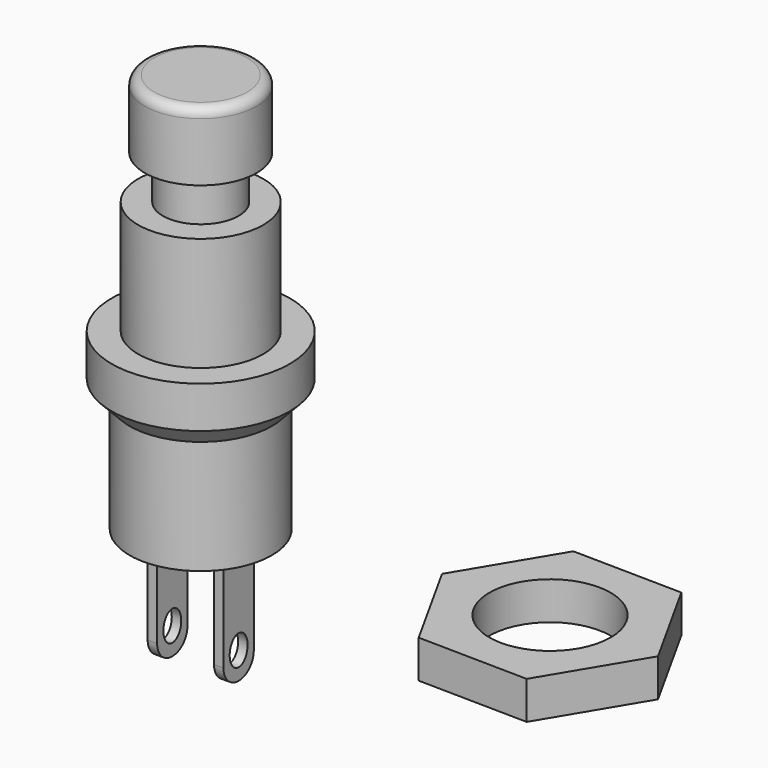
from build123d import *

# Parameters (mm, degrees)
F0_R      = 3.75
F0_W      = 0.5
F0_H      = 2
F1_DEPTH  = 6
F3_R      = 4.7
F1_FACE_R = 3.75
F5_DEPTH  = 2.2
F6_R      = 3.3
F7_DEPTH  = 6
F8_R      = 2
F9_DEPTH  = 2.3
F10_R     = 2.95
F11_DEPTH = 3.6
F12_R     = 0.5
F13_DEPTH = 6.4
F15_DEPTH = 6.7010001
F16_R     = 0.99999
F0_R_2    = 3.2
F17_DEPTH = 2


# Not quite as in the source:
# - a fillet or chamfer is up to 0.001 mm smaller than in the source, because OpenCascade refuses the exact size


with BuildPart() as f1:
    # F0 (on Top) → F1 (new body)
    with BuildSketch(Plane.XY):
        Circle(F0_R)
        with Locations((-1.75, 0)):
            Rectangle(F0_W, F0_H, mode=Mode.SUBTRACT)
        with Locations((1.75, 0)):
            Rectangle(F0_W, F0_H, mode=Mode.SUBTRACT)
        with Locations((-1.75, 0)):
            Rectangle(F0_W, F0_H)
        with Locations((1.75, 0)):
            Rectangle(F0_W, F0_H)
    extrude(amount=F1_DEPTH)

    # F3 (on offset) → F4 section 0
    with BuildSketch(Plane.XY.offset(7)):
        Circle(F3_R)
    # F1_face (on face) → F4 section 1
    with BuildSketch(Plane.XY.offset(6)):
        Circle(F1_FACE_R)
    loft()

    # F3 (on offset) → F5 (join)
    with BuildSketch(Plane.XY.offset(7)):
        Circle(F3_R)
    extrude(amount=F5_DEPTH)

    # F6 (on face) → F7 (join)
    with BuildSketch(Plane.XY.offset(9.2)):
        Circle(F6_R)
    extrude(amount=F7_DEPTH)

    # F8 (on face) → F9 (join)
    with BuildSketch(Plane.XY.offset(15.2)):
        Circle(F8_R)
    extrude(amount=F9_DEPTH)

    # F0 (on Top) → F13 (join)
    with BuildSketch(Plane.XY):
        with Locations((-1.75, 0)):
            Rectangle(F0_W, F0_H)
        with Locations((1.75, 0)):
            Rectangle(F0_W, F0_H)
    extrude(amount=-F13_DEPTH)

    # F14 (on face) → F15 (cut, through all)
    with BuildSketch(Plane.YZ.offset(2)):
        with BuildLine():
            add(Edge.make_bspline(
                [(0, -5.7707964443), (1.0216056149, -5.7707964443), (0.5108028075, -4.5781605877), (0, -3.3855247311), (-0.5108028075, -4.5781605877), (-1.0216056149, -5.7707964443), (0, -5.7707964443)],
                knots=[0, 0, 0, 2.0943951024, 2.0943951024, 4.1887902048, 4.1887902048, 6.2831853072, 6.2831853072, 6.2831853072], degree=2, weights=[1, 0.5, 1, 0.5, 1, 0.5, 1]))
        make_face()
    extrude(amount=-F15_DEPTH, mode=Mode.SUBTRACT)

    # F16 (radius 1 in the source; OpenCascade refuses exactly that, so slightly less here)
    f16_edges = [f1.edges().sort_by_distance(p)[0] for p in [
        (1.75, 1, -6.4),
        (1.75, -1, -6.4),
        (-1.75, 1, -6.4),
        (-1.75, -1, -6.4),
    ]]
    fillet(f16_edges, radius=F16_R)


with BuildPart() as f11:
    # F10 (on face) → F11 (new body)
    with BuildSketch(Plane.XY.offset(17.5)):
        Circle(F10_R)
    extrude(amount=F11_DEPTH)

    # F12
    f12_edges = [f11.edges().sort_by_distance(p)[0] for p in [
        (-2.95, 0, 21.1),
    ]]
    fillet(f12_edges, radius=F12_R)


with BuildPart() as f17:
    # F0 (on Top) → F17 (new body)
    with BuildSketch(Plane.XY):
        Polygon((24.2037526902, -0.0936588947), (21.3984921896, 4.9525126102), (15.6257492242, 5.0461715049), (12.6582667593, 0.0936588947), (15.4635272599, -4.9525126102), (21.2362702253, -5.0461715049), align=None)
        with Locations((18.4310097247, 0)):
            Circle(F0_R_2, mode=Mode.SUBTRACT)
    extrude(amount=F17_DEPTH)


solid = Compound([f1.part, f11.part, f17.part])
